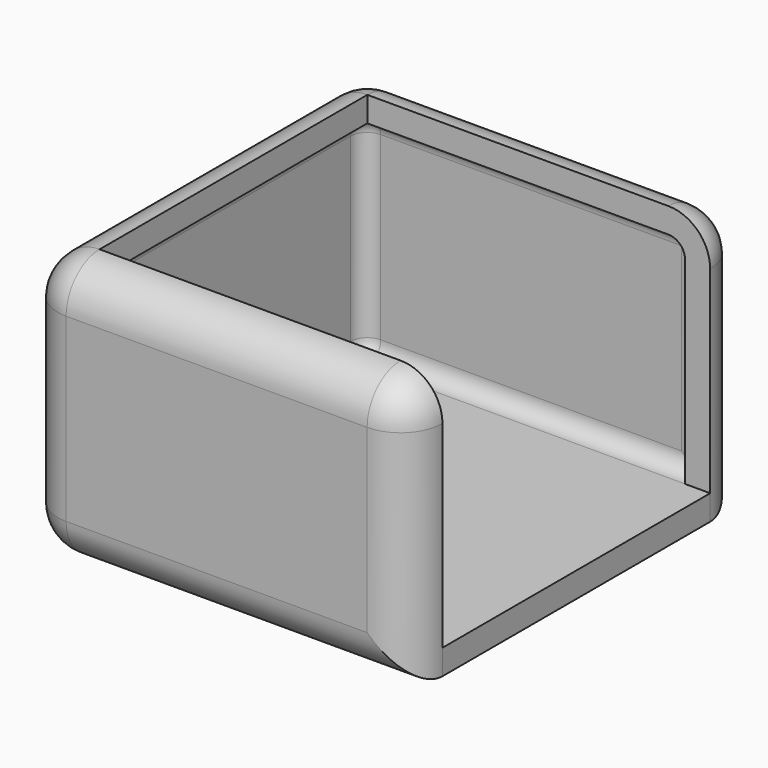
from build123d import *

# Parameters (mm, degrees)
F0_W     = 116.7918927968
F0_H     = 80.2520625293
F1_DEPTH = 63.5
F2_R     = 12.7
F3_T     = 7.62


# Not quite as in the source:
# - a shell that OpenCascade refuses in one call is made with other operations: the cavity is built on its own and cut out


with BuildPart() as f1:
    # F0 (on Front) → F1 (new body, symmetric)
    with BuildSketch(Plane.XZ):
        with Locations((1.3399217278, 3.6678072065)):
            Rectangle(F0_W, F0_H)
    extrude(amount=F1_DEPTH, both=True)

    # F2
    f2_edges = [f1.edges().sort_by_distance(p)[0] for p in [
        (-57.056025, 0, 43.793838),
        (1.339922, 63.5, 43.793838),
        (59.735868, 0, 43.793838),
        (-57.056025, -63.5, 3.667807),
        (-57.056025, 63.5, 3.667807),
        (59.735868, -63.5, 3.667807),
        (59.735868, 63.5, 3.667807),
        (1.339922, 63.5, -36.458224),
        (1.339922, -63.5, -36.458224),
        (-57.056025, 0, -36.458224),
        (1.339922, -63.5, 43.793838),
    ]]
    fillet(f2_edges, radius=F2_R)

    # F3: shell of thickness 7.62, made by hand


with BuildPart() as f3_core1:
    # F3_t2: copy of F1
    add(f1.part)

    # the walls: a layer under each face that stays
    f3_faces = [f3_core1.faces().sort_by_distance(p)[0] for p in [
        (-53.3362807917, 0, 40.0740945922),
        (1.3399217278, 59.7802561211, 40.0740945922),
        (1.3399217278, -59.7802561211, 40.0740945922),
        (-50.7060246706, 59.7802561211, 37.4438384712),
        (-50.7060246706, -59.7802561211, 37.4438384712),
        (-57.0560246706, 0, 3.6678072065),
        (56.0161242472, 57.15, 37.4438384712),
        (1.3399217278, 63.5, 3.6678072065),
        (53.3858681262, -59.7802561211, 37.4438384712),
        (1.3399217278, -63.5, 3.6678072065),
        (-53.3362807917, 59.7802561211, 3.6678072065),
        (-53.3362807917, -59.7802561211, 3.6678072065),
        (-53.3362807917, 0, -32.7384801792),
        (56.0161242472, 59.7802561211, -2.6821927935),
        (7.6899217278, 59.7802561211, -32.7384801792),
        (56.0161240867, -59.7802562816, -2.6821927935),
        (7.6899217278, -59.7802562816, -32.7384800187),
        (7.6899217278, 0, -36.4582240582),
        (-50.7060246706, 57.15, -32.7384801792),
        (-50.7060246706, -57.15, -32.7384801792),
    ]]
    thicken(f3_faces, amount=-F3_T, mode=Mode.SUBTRACT)


with BuildPart() as f1_1:
    add(f1.part)

    # what is left inside the walls is the cavity
    f3_cavity = [f3_core1.part.solids().sort_by_distance(p)[0] for p in [
        (7.689922, 16.933333, -28.762024),
    ]]
    add(f3_cavity, mode=Mode.SUBTRACT)


solid = f1_1.part
